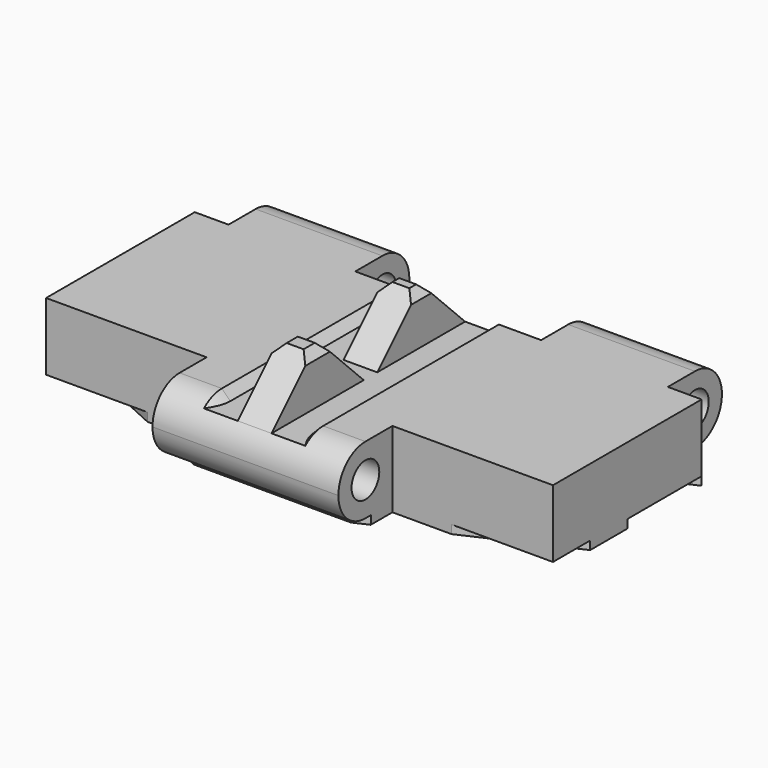
from build123d import *

# Parameters (mm, degrees)
F0_W      = 30
F0_H      = 15
F1_DEPTH  = 4.5
F3_DEPTH  = 30
F4_W      = 9.5
F4_H      = 2
F4_W_2    = 2
F4_W_3    = 11
F5_DEPTH  = 25
F6_R      = 1.025
F7_DEPTH  = 30
F8_W      = 9.5
F8_H      = 2
F9_DEPTH  = 25
F10_W     = 11
F10_H     = 2
F11_DEPTH = 25
F12_W     = 2
F12_H     = 2
F13_DEPTH = 25
F15_DEPTH = 0.5
F16_W     = 5
F16_H     = 13
F16_H_2   = 3.8236103207
F17_DEPTH = 0.5
F18_W     = 2
F18_H     = 14.3228756555
F19_DEPTH = 3
F20_SIZE  = 2.99999
F21_SIZE  = 3
F22_SIZE  = 0.5
F23_SIZE  = 0.49999
F25_DEPTH = 3


# Not quite as in the source:
# - a fillet or chamfer is up to 0.001 mm smaller than in the source, because OpenCascade refuses the exact size
# - a feature names something its author has since deleted; it is built from what else it names


with BuildPart() as f1:
    # F0 (on Top) → F1 (new body)
    with BuildSketch(Plane.XY):
        Rectangle(F0_W, F0_H)
    extrude(amount=F1_DEPTH)

    # F2 (on face) → F3 (join)
    with BuildSketch(Plane(origin=(-15, 0, 0), x_dir=(0, -1, 0), z_dir=(-1, 0, 0))):
        with BuildLine():
            ThreePointArc((-7.5, 0.5), (-6.0857864376, 1.0857864376), (-5.5, 2.5))
            ThreePointArc((-5.5, 2.5), (-6.0857864376, 3.9142135624), (-7.5, 4.5))
            Line((-7.5, 4.5), (-7.5, 0.5))
        make_face()
        with BuildLine():
            Line((-7.5, 0.5), (-7.5, 4.5))
            ThreePointArc((-7.5, 4.5), (-9.5, 2.5), (-7.5, 0.5))
        make_face()
        with BuildLine():
            ThreePointArc((9.5, 2.5), (8.9142135624, 3.9142135624), (7.5, 4.5))
            Line((7.5, 4.5), (7.5, 0.5))
            ThreePointArc((7.5, 0.5), (8.9142135624, 1.0857864376), (9.5, 2.5))
        make_face()
    extrude(amount=-F3_DEPTH)

    # F4 (on face) → F5 (cut)
    with BuildSketch(Plane.XY.offset(4.5)):
        with Locations((-10.25, -8.5)):
            Rectangle(F4_W, F4_H)
        with Locations((10.25, -8.5)):
            Rectangle(F4_W, F4_H)
        with Locations((-14, 8.5)):
            Rectangle(F4_W_2, F4_H)
        with Locations((14, 8.5)):
            Rectangle(F4_W_2, F4_H)
        with Locations((0, 8.5)):
            Rectangle(F4_W_3, F4_H)
    extrude(amount=-F5_DEPTH, mode=Mode.SUBTRACT)

    # F6 (on face) → F7 (cut)
    with BuildSketch(Plane.YZ.offset(15)):
        with Locations((-7.5, 2.5)):
            Circle(F6_R)
        with Locations((7.5, 2.5)):
            Circle(F6_R)
    extrude(amount=-F7_DEPTH, mode=Mode.SUBTRACT)

    # F8 (on face) → F9 (cut)
    with BuildSketch(Plane.XY.offset(4.5)):
        with Locations((-10.25, -6.5)):
            Rectangle(F8_W, F8_H)
        with Locations((10.25, -6.5)):
            Rectangle(F8_W, F8_H)
    extrude(amount=-F9_DEPTH, mode=Mode.SUBTRACT)

    # F10 (on face) → F11 (cut)
    with BuildSketch(Plane.XY.offset(4.5)):
        with Locations((0, 6.5)):
            Rectangle(F10_W, F10_H)
    extrude(amount=-F11_DEPTH, mode=Mode.SUBTRACT)

    # F12 (on face) → F13 (cut)
    with BuildSketch(Plane.XY.offset(4.5)):
        with Locations((-14, 6.5)):
            Rectangle(F12_W, F12_H)
        with Locations((14, 6.5)):
            Rectangle(F12_W, F12_H)
    extrude(amount=-F13_DEPTH, mode=Mode.SUBTRACT)

    # F14 (on face) → F15 (cut)
    with BuildSketch(Plane(origin=(0, 0, 0), x_dir=(1, 0, 0), z_dir=(0, 0, -1))):
        Polygon((3, 5.5), (0, 5.5), (-3, 5.5), (-15, 0), (-15, -5.5), (-3, 0), (3, 0), (15, -5.5), (15, 0), align=None)
        Polygon((-15, 5.5), (-15, 2.75), (-9, 5.5), align=None)
        Polygon((9, 5.5), (15, 2.75), (15, 5.5), align=None)
        Polygon((-3, -2.75), (-13, -7.3333333333), (-13, -7.5), (-5.5, -7.5), (-5.5, -5.5), (5.5, -5.5), (5.5, -7.5), (13, -7.5), (13, -7.3333333333), (3, -2.75), align=None)
        Polygon((-5.5, 7.5), (-5.5, 7.1041666667), (-4.6363636364, 7.5), align=None)
        Polygon((4.6363636364, 7.5), (5.5, 7.1041666667), (5.5, 7.5), align=None)
    extrude(amount=-F15_DEPTH, mode=Mode.SUBTRACT)

    # F16 (on face) → F17 (cut)
    with BuildSketch(Plane.XY.offset(4.5)):
        with Locations((0, -1)):
            Rectangle(F16_W, F16_H)
        with Locations((0, -9.4118051603)):
            Rectangle(F16_W, F16_H_2)
    extrude(amount=-F17_DEPTH, mode=Mode.SUBTRACT)

    # F18 (on face) → F19 (join)
    with BuildSketch(Plane.XY.offset(4)):
        with Locations((0, -1.6614378278)):
            Rectangle(F18_W, F18_H)
    extrude(amount=F19_DEPTH)

    # F20 (size 3 in the source; OpenCascade refuses exactly that, so slightly less here)
    f20_edges = [f1.edges().sort_by_distance(p)[0] for p in [
        (0, -8.822876, 7),
    ]]
    chamfer(f20_edges, length=F20_SIZE)

    # F21
    f21_edges = [f1.edges().sort_by_distance(p)[0] for p in [
        (0, 5.5, 7),
    ]]
    chamfer(f21_edges, length=F21_SIZE)

    # F22
    f22_edges = [f1.edges().sort_by_distance(p)[0] for p in [
        (-1, -1.661443, 7),
        (1, -1.661443, 7),
    ]]
    chamfer(f22_edges, length=F22_SIZE)

    # F23 (size 0.5 in the source; OpenCascade refuses exactly that, so slightly less here)
    f23_edges = [f1.edges().sort_by_distance(p)[0] for p in [
        (2.5, -1, 4.5),
        (-2.5, -1, 4.5),
    ]]
    chamfer(f23_edges, length=F23_SIZE)

    # F24 (on face) → F25 (cut)
    with BuildSketch(Plane.YZ.offset(1)):
        Polygon((-5, 7), (-4.5, 6.5), (1.5, 6.5), (2, 7), align=None)
        Polygon((-4.5, 6.5), (-2, 4), (-1.5, 4), (-1, 4), (1.5, 6.5), align=None)
    extrude(amount=-F25_DEPTH, mode=Mode.SUBTRACT)


solid = f1.part
